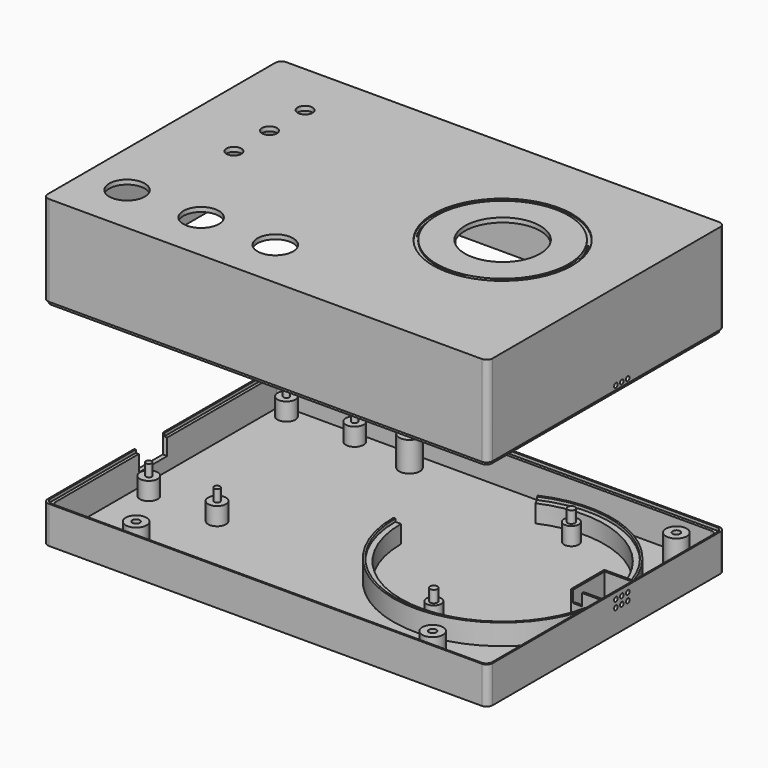
from build123d import *

# Parameters (mm, degrees)
F1_DEPTH  = 6
F0_R      = 2.5
F0_R_2    = 1.25
F0_R_3    = 3
F0_R_4    = 1
F0_W      = 3
F0_H      = 0.7
F2_DEPTH  = 10
F3_DEPTH  = 10
F0_R_5    = 3.5
F4_DEPTH  = 10
F5_DEPTH  = 4.5
F6_DEPTH  = 11
F7_DEPTH  = 7
F8_START  = 7.5
F8_DEPTH  = 2.5
F9_DEPTH  = 1.5
F10_R     = 2
F14_DEPTH = 30
F13_R     = 3.5
F15_DEPTH = 29
F13_R_2   = 2
F16_DEPTH = 7
F13_R_3   = 6
F13_R_4   = 2.5
F13_R_5   = 23.495
F17_DEPTH = 1.5
F13_R_6   = 12.7
F18_DEPTH = 1
F19_D     = 1.6
F19_DEPTH = 30.001
F20_D     = 1.6
F20_DEPTH = 30.001
F22_R     = 2
F23_DEPTH = 28
F24_DEPTH = 27
F26_R     = 0.75
F27_DEPTH = 1.5


# Not quite as in the source:
# - a feature of the source that left no trace in its solid (it failed there, or was rolled back) is left out
# - a feature names something its author has since deleted; it is built from what else it names


with BuildPart() as f1:
    # F0 (on Top) → F1 (new body)
    with BuildSketch(Plane.XY):
        with BuildLine():
            ThreePointArc((-14.0198845395, 31.2929215239), (15.59063064, 30.5407324118), (33.567902824, 7))
            Line((33.567902824, 7), (35.5116604089, 7))
            ThreePointArc((35.5116604089, 7), (16.6332395549, 32.1467473768), (-14.798767014, 33.0314171641))
            Line((-14.798767014, 33.0314171641), (-14.0198845395, 31.2929215239))
        make_face()
    extrude(amount=F1_DEPTH)



with BuildPart() as f1b:
    # F0 (on Top) → F1, piece 2 (new body)
    with BuildSketch(Plane.XY):
        with BuildLine():
            Line((-34.29, 0), (-36.195, 0))
            ThreePointArc((-36.195, 0), (-3.5166373497, -36.0237600307), (35.5116604089, -7))
            Line((35.5116604089, -7), (33.567902824, -7))
            ThreePointArc((33.567902824, -7), (-3.518573018, -34.1089979905), (-34.29, 0))
        make_face()
    extrude(amount=F1_DEPTH)


with BuildPart() as f1c:
    # F0 (on Top) → F1, piece 3 (new body)
    with BuildSketch(Plane.XY):
        with Locations((0, -29)):
            Circle(F0_R)
        with Locations((0, -29)):
            Circle(F0_R_2, mode=Mode.SUBTRACT)
    extrude(amount=F1_DEPTH)

    # F0 (on Top) → F2, piece 2 (join)
    with BuildSketch(Plane.XY):
        with Locations((0, -29)):
            Circle(F0_R_2)
    extrude(amount=F2_DEPTH)


with BuildPart() as f1d:
    # F0 (on Top) → F1, piece 4 (new body)
    with BuildSketch(Plane.XY):
        with Locations((0, 29)):
            Circle(F0_R)
        with Locations((0, 29)):
            Circle(F0_R_2, mode=Mode.SUBTRACT)
    extrude(amount=F1_DEPTH)

    # F0 (on Top) → F2 (join)
    with BuildSketch(Plane.XY):
        with Locations((0, 29)):
            Circle(F0_R_2)
    extrude(amount=F2_DEPTH)


with BuildPart() as f1e:
    # F0 (on Top) → F1, piece 5 (new body)
    with BuildSketch(Plane.XY):
        with Locations((-80.305, 38.0003526509)):
            Circle(F0_R_3)
        with Locations((-80.305, 38.0003526509)):
            Circle(F0_R_4, mode=Mode.SUBTRACT)
    extrude(amount=F1_DEPTH)

    # F0 (on Top) → F2, piece 4 (join)
    with BuildSketch(Plane.XY):
        with Locations((-80.305, 38.0003526509)):
            Circle(F0_R_4)
    extrude(amount=F2_DEPTH)


with BuildPart() as f1f:
    # F0 (on Top) → F1, piece 6 (new body)
    with BuildSketch(Plane.XY):
        with Locations((-103.305, 38.0003526509)):
            Circle(F0_R_3)
        with Locations((-103.305, 38.0003526509)):
            Circle(F0_R_4, mode=Mode.SUBTRACT)
    extrude(amount=F1_DEPTH)

    # F0 (on Top) → F2, piece 3 (join)
    with BuildSketch(Plane.XY):
        with Locations((-103.305, 38.0003526509)):
            Circle(F0_R_4)
    extrude(amount=F2_DEPTH)


with BuildPart() as f1g:
    # F0 (on Top) → F1, piece 7 (new body)
    with BuildSketch(Plane.XY):
        with Locations((-80.305, -19.9996473491)):
            Circle(F0_R_3)
        with Locations((-80.305, -19.9996473491)):
            Circle(F0_R_4, mode=Mode.SUBTRACT)
    extrude(amount=F1_DEPTH)

    # F0 (on Top) → F2, piece 5 (join)
    with BuildSketch(Plane.XY):
        with Locations((-80.305, -19.9996473491)):
            Circle(F0_R_4)
    extrude(amount=F2_DEPTH)


with BuildPart() as f1h:
    # F0 (on Top) → F1, piece 8 (new body)
    with BuildSketch(Plane.XY):
        with Locations((-103.305, -19.9996473491)):
            Circle(F0_R_3)
        with Locations((-103.305, -19.9996473491)):
            Circle(F0_R_4, mode=Mode.SUBTRACT)
    extrude(amount=F1_DEPTH)

    # F0 (on Top) → F2, piece 6 (join)
    with BuildSketch(Plane.XY):
        with Locations((-103.305, -19.9996473491)):
            Circle(F0_R_4)
    extrude(amount=F2_DEPTH)


with BuildPart() as f1i:
    # F0 (on Top) → F1, piece 9 (new body)
    with BuildSketch(Plane.XY):
        with Locations((30.895, -6.65)):
            Rectangle(F0_W, F0_H)
    extrude(amount=F1_DEPTH)


with BuildPart() as f1j:
    # F0 (on Top) → F1, piece 10 (new body)
    with BuildSketch(Plane.XY):
        Polygon((-96.805, 42.0003526509), (-82.805, 42.0003526509), (-82.805, 43.0003526509), (-82.805, 43.5003526509), (-96.805, 43.5003526509), (-96.805, 43.0003526509), align=None)
    extrude(amount=F1_DEPTH)


with BuildPart() as f1_1:
    add(f1.part)

    add(f1b.part)  # F3 merges F1b

    add(f1i.part)  # F3 merges F1i
    # F0 (on Top) → F3 (join)
    with BuildSketch(Plane.XY):
        Polygon((28.695, -7), (29.395, -7), (29.395, -6.3), (29.395, 6.3), (38.695, 6.3), (38.695, 7), (36.1586628624, 7), (35.5116604089, 7), (33.567902824, 7), (28.695, 7), align=None)
        Polygon((33.567902824, -7), (35.5116604089, -7), (36.1586628624, -7), (38.695, -7), (38.695, -6.3), (32.395, -6.3), (32.395, -7), align=None)
    extrude(amount=F3_DEPTH)


    add(f1j.part)  # F4 merges F1j
    # F0 (on Top) → F4 (join)
    with BuildSketch(Plane.XY):
        Polygon((38.695, -6.3), (38.695, -7), (38.695, -54.9996473491), (-108.305, -54.9996473491), (-108.305, -17.9996473491), (-109.305, -17.9996473491), (-109.305, -55.9996473491), (39.695, -55.9996473491), (39.695, 43.0003526509), (-82.805, 43.0003526509), (-82.805, 42.0003526509), (38.695, 42.0003526509), (38.695, 7), (38.695, 6.3), align=None)
        Polygon((-109.305, -5.9996473491), (-108.305, -5.9996473491), (-108.305, 42.0003526509), (-96.805, 42.0003526509), (-96.805, 43.0003526509), (-109.305, 43.0003526509), align=None)
    extrude(amount=F4_DEPTH)

    # F0 (on Top) → F5 (join)
    with BuildSketch(Plane.XY):
        Polygon((-109.305, -17.9996473491), (-108.305, -17.9996473491), (-108.305, -5.9996473491), (-109.305, -5.9996473491), (-109.805, -5.9996473491), (-109.805, -17.9996473491), align=None)
    extrude(amount=F5_DEPTH)

    # F0 (on Top) → F6 (join)
    with BuildSketch(Plane.XY):
        Polygon((-109.305, -55.9996473491), (-109.305, -17.9996473491), (-109.805, -17.9996473491), (-109.805, -56.4996473491), (40.195, -56.4996473491), (40.195, 43.5003526509), (-82.805, 43.5003526509), (-82.805, 43.0003526509), (39.695, 43.0003526509), (39.695, -55.9996473491), align=None)
        Polygon((-109.805, -5.9996473491), (-109.305, -5.9996473491), (-109.305, 43.0003526509), (-96.805, 43.0003526509), (-96.805, 43.5003526509), (-109.805, 43.5003526509), align=None)
    extrude(amount=F6_DEPTH)

    # F0 (on Top) → F7 (join)
    with BuildSketch(Plane.XY):
        with BuildLine():
            Line((35.5116604089, 7), (36.1586628624, 7))
            ThreePointArc((36.1586628624, 7), (16.9805930381, 32.6819271169), (-15.0583945054, 33.6109157108))
            Line((-15.0583945054, 33.6109157108), (-14.798767014, 33.0314171641))
            ThreePointArc((-14.798767014, 33.0314171641), (16.6332395549, 32.1467473768), (35.5116604089, 7))
        make_face()
        with BuildLine():
            ThreePointArc((35.5116604089, -7), (-3.5166373497, -36.0237600307), (-36.195, 0))
            Line((-36.195, 0), (-36.83, 0))
            ThreePointArc((-36.83, 0), (-3.516059355, -36.6617815526), (36.1586628624, -7))
            Line((36.1586628624, -7), (35.5116604089, -7))
        make_face()
    extrude(amount=F7_DEPTH)


    add(f1c.part)  # F9 merges F1c

    add(f1d.part)  # F9 merges F1d

    add(f1e.part)  # F9 merges F1e

    add(f1f.part)  # F9 merges F1f

    add(f1g.part)  # F9 merges F1g

    add(f1h.part)  # F9 merges F1h


with BuildPart() as f3:
    # F0 (on Top) → F3, piece 2 (new body)
    with BuildSketch(Plane.XY):
        with Locations((15.195, -48.4996473491)):
            Circle(F0_R_5)
        with Locations((15.195, -48.4996473491)):
            Circle(F0_R, mode=Mode.SUBTRACT)
    extrude(amount=F3_DEPTH)

    # F0 (on Top) → F8, piece 3 (join)
    with BuildSketch(Plane.XY.offset(F8_START)):
        with Locations((15.195, -48.4996473491)):
            Circle(F0_R)
        with Locations((15.195, -48.4996473491)):
            Circle(F0_R_2, mode=Mode.SUBTRACT)
    extrude(amount=F8_DEPTH)


with BuildPart() as f3b:
    # F0 (on Top) → F3, piece 3 (new body)
    with BuildSketch(Plane.XY):
        with Locations((30.195, 35.5003526509)):
            Circle(F0_R_5)
        with Locations((30.195, 35.5003526509)):
            Circle(F0_R, mode=Mode.SUBTRACT)
    extrude(amount=F3_DEPTH)

    # F0 (on Top) → F8, piece 4 (join)
    with BuildSketch(Plane.XY.offset(F8_START)):
        with Locations((30.195, 35.5003526509)):
            Circle(F0_R)
        with Locations((30.195, 35.5003526509)):
            Circle(F0_R_2, mode=Mode.SUBTRACT)
    extrude(amount=F8_DEPTH)


with BuildPart() as f3c:
    # F0 (on Top) → F3, piece 4 (new body)
    with BuildSketch(Plane.XY):
        with Locations((-84.805, -48.4996473491)):
            Circle(F0_R_5)
        with Locations((-84.805, -48.4996473491)):
            Circle(F0_R, mode=Mode.SUBTRACT)
    extrude(amount=F3_DEPTH)

    # F0 (on Top) → F8 (join)
    with BuildSketch(Plane.XY.offset(F8_START)):
        with Locations((-84.805, -48.4996473491)):
            Circle(F0_R)
        with Locations((-84.805, -48.4996473491)):
            Circle(F0_R_2, mode=Mode.SUBTRACT)
    extrude(amount=F8_DEPTH)


with BuildPart() as f3d:
    # F0 (on Top) → F3, piece 5 (new body)
    with BuildSketch(Plane.XY):
        with Locations((-59.805, 35.5003526509)):
            Circle(F0_R_5)
        with Locations((-59.805, 35.5003526509)):
            Circle(F0_R, mode=Mode.SUBTRACT)
    extrude(amount=F3_DEPTH)

    # F0 (on Top) → F8, piece 2 (join)
    with BuildSketch(Plane.XY.offset(F8_START)):
        with Locations((-59.805, 35.5003526509)):
            Circle(F0_R)
        with Locations((-59.805, 35.5003526509)):
            Circle(F0_R_2, mode=Mode.SUBTRACT)
    extrude(amount=F8_DEPTH)


with BuildPart() as f1_2:
    add(f1_1.part)

    add(f3.part)  # F9 merges F3

    add(f3b.part)  # F9 merges F3b

    add(f3c.part)  # F9 merges F3c

    add(f3d.part)  # F9 merges F3d
    # F0 (on Top) → F9 (join)
    with BuildSketch(Plane.XY):
        Polygon((-109.305, -55.9996473491), (-109.305, -17.9996473491), (-109.805, -17.9996473491), (-109.805, -56.4996473491), (40.195, -56.4996473491), (40.195, 43.5003526509), (-82.805, 43.5003526509), (-82.805, 43.0003526509), (39.695, 43.0003526509), (39.695, -55.9996473491), align=None)
        Polygon((38.695, -6.3), (38.695, -7), (38.695, -54.9996473491), (-108.305, -54.9996473491), (-108.305, -17.9996473491), (-109.305, -17.9996473491), (-109.305, -55.9996473491), (39.695, -55.9996473491), (39.695, 43.0003526509), (-82.805, 43.0003526509), (-82.805, 42.0003526509), (38.695, 42.0003526509), (38.695, 7), (38.695, 6.3), align=None)
        Polygon((-109.305, -17.9996473491), (-108.305, -17.9996473491), (-108.305, -5.9996473491), (-109.305, -5.9996473491), (-109.805, -5.9996473491), (-109.805, -17.9996473491), align=None)
        Polygon((-109.805, -5.9996473491), (-109.305, -5.9996473491), (-109.305, 43.0003526509), (-96.805, 43.0003526509), (-96.805, 43.5003526509), (-109.805, 43.5003526509), align=None)
        Polygon((-109.305, -5.9996473491), (-108.305, -5.9996473491), (-108.305, 42.0003526509), (-96.805, 42.0003526509), (-96.805, 43.0003526509), (-109.305, 43.0003526509), align=None)
        Polygon((-96.805, 42.0003526509), (-82.805, 42.0003526509), (-82.805, 43.0003526509), (-82.805, 43.5003526509), (-96.805, 43.5003526509), (-96.805, 43.0003526509), align=None)
        with BuildLine():
            Line((-36.83, 0), (-36.195, 0))
            Line((-36.195, 0), (-34.29, 0))
            ThreePointArc((-34.29, 0), (-3.518573018, -34.1089979905), (33.567902824, -7))
            Line((33.567902824, -7), (32.395, -7))
            Line((32.395, -7), (29.395, -7))
            Line((29.395, -7), (28.695, -7))
            Line((28.695, -7), (28.695, 7))
            Line((28.695, 7), (33.567902824, 7))
            ThreePointArc((33.567902824, 7), (15.59063064, 30.5407324118), (-14.0198845395, 31.2929215239))
            Line((-14.0198845395, 31.2929215239), (-14.798767014, 33.0314171641))
            Line((-14.798767014, 33.0314171641), (-15.0583945054, 33.6109157108))
            ThreePointArc((-15.0583945054, 33.6109157108), (16.9805930381, 32.6819271169), (36.1586628624, 7))
            Line((36.1586628624, 7), (38.695, 7))
            Line((38.695, 7), (38.695, 42.0003526509))
            Line((38.695, 42.0003526509), (-82.805, 42.0003526509))
            Line((-82.805, 42.0003526509), (-96.805, 42.0003526509))
            Line((-96.805, 42.0003526509), (-108.305, 42.0003526509))
            Line((-108.305, 42.0003526509), (-108.305, -5.9996473491))
            Line((-108.305, -5.9996473491), (-108.305, -17.9996473491))
            Line((-108.305, -17.9996473491), (-108.305, -54.9996473491))
            Line((-108.305, -54.9996473491), (38.695, -54.9996473491))
            Line((38.695, -54.9996473491), (38.695, -7))
            Line((38.695, -7), (36.1586628624, -7))
            ThreePointArc((36.1586628624, -7), (-3.516059355, -36.6617815526), (-36.83, 0))
        make_face()
        with Locations((-84.805, -48.4996473491)):
            Circle(F0_R_5, mode=Mode.SUBTRACT)
        with Locations((-103.305, -19.9996473491)):
            Circle(F0_R_3, mode=Mode.SUBTRACT)
        with Locations((-80.305, -19.9996473491)):
            Circle(F0_R_3, mode=Mode.SUBTRACT)
        with Locations((15.195, -48.4996473491)):
            Circle(F0_R_5, mode=Mode.SUBTRACT)
        with Locations((0, -29)):
            Circle(F0_R, mode=Mode.SUBTRACT)
        with Locations((-103.305, 38.0003526509)):
            Circle(F0_R_3, mode=Mode.SUBTRACT)
        with Locations((-80.305, 38.0003526509)):
            Circle(F0_R_3, mode=Mode.SUBTRACT)
        with Locations((-59.805, 35.5003526509)):
            Circle(F0_R_5, mode=Mode.SUBTRACT)
        with Locations((0, 29)):
            Circle(F0_R, mode=Mode.SUBTRACT)
        with Locations((30.195, 35.5003526509)):
            Circle(F0_R_5, mode=Mode.SUBTRACT)
        with Locations((-103.305, 38.0003526509)):
            Circle(F0_R_3)
        with Locations((-103.305, 38.0003526509)):
            Circle(F0_R_4, mode=Mode.SUBTRACT)
        with Locations((-103.305, 38.0003526509)):
            Circle(F0_R_4)
        with Locations((-80.305, 38.0003526509)):
            Circle(F0_R_3)
        with Locations((-80.305, 38.0003526509)):
            Circle(F0_R_4, mode=Mode.SUBTRACT)
        with Locations((-80.305, 38.0003526509)):
            Circle(F0_R_4)
        with Locations((-59.805, 35.5003526509)):
            Circle(F0_R_5)
        with Locations((-59.805, 35.5003526509)):
            Circle(F0_R, mode=Mode.SUBTRACT)
        with Locations((-84.805, -48.4996473491)):
            Circle(F0_R_5)
        with Locations((-84.805, -48.4996473491)):
            Circle(F0_R, mode=Mode.SUBTRACT)
        with Locations((-103.305, -19.9996473491)):
            Circle(F0_R_3)
        with Locations((-103.305, -19.9996473491)):
            Circle(F0_R_4, mode=Mode.SUBTRACT)
        with Locations((-103.305, -19.9996473491)):
            Circle(F0_R_4)
        with Locations((-80.305, -19.9996473491)):
            Circle(F0_R_3)
        with Locations((-80.305, -19.9996473491)):
            Circle(F0_R_4, mode=Mode.SUBTRACT)
        with Locations((-80.305, -19.9996473491)):
            Circle(F0_R_4)
        with Locations((0, 29)):
            Circle(F0_R)
        with Locations((0, 29)):
            Circle(F0_R_2, mode=Mode.SUBTRACT)
        with Locations((0, 29)):
            Circle(F0_R_2)
        with BuildLine():
            ThreePointArc((-14.0198845395, 31.2929215239), (15.59063064, 30.5407324118), (33.567902824, 7))
            Line((33.567902824, 7), (35.5116604089, 7))
            ThreePointArc((35.5116604089, 7), (16.6332395549, 32.1467473768), (-14.798767014, 33.0314171641))
            Line((-14.798767014, 33.0314171641), (-14.0198845395, 31.2929215239))
        make_face()
        with BuildLine():
            Line((35.5116604089, 7), (36.1586628624, 7))
            ThreePointArc((36.1586628624, 7), (16.9805930381, 32.6819271169), (-15.0583945054, 33.6109157108))
            Line((-15.0583945054, 33.6109157108), (-14.798767014, 33.0314171641))
            ThreePointArc((-14.798767014, 33.0314171641), (16.6332395549, 32.1467473768), (35.5116604089, 7))
        make_face()
        with BuildLine():
            Line((-34.29, 0), (-36.195, 0))
            ThreePointArc((-36.195, 0), (-3.5166373497, -36.0237600307), (35.5116604089, -7))
            Line((35.5116604089, -7), (33.567902824, -7))
            ThreePointArc((33.567902824, -7), (-3.518573018, -34.1089979905), (-34.29, 0))
        make_face()
        with BuildLine():
            ThreePointArc((35.5116604089, -7), (-3.5166373497, -36.0237600307), (-36.195, 0))
            Line((-36.195, 0), (-36.83, 0))
            ThreePointArc((-36.83, 0), (-3.516059355, -36.6617815526), (36.1586628624, -7))
            Line((36.1586628624, -7), (35.5116604089, -7))
        make_face()
        with Locations((30.195, 35.5003526509)):
            Circle(F0_R_5)
        with Locations((30.195, 35.5003526509)):
            Circle(F0_R, mode=Mode.SUBTRACT)
        Polygon((28.695, -7), (29.395, -7), (29.395, -6.3), (29.395, 6.3), (38.695, 6.3), (38.695, 7), (36.1586628624, 7), (35.5116604089, 7), (33.567902824, 7), (28.695, 7), align=None)
        Polygon((32.395, -6.3), (38.695, -6.3), (38.695, 6.3), (29.395, 6.3), (29.395, -6.3), align=None)
        Polygon((33.567902824, -7), (35.5116604089, -7), (36.1586628624, -7), (38.695, -7), (38.695, -6.3), (32.395, -6.3), (32.395, -7), align=None)
        with Locations((30.895, -6.65)):
            Rectangle(F0_W, F0_H)
        with Locations((0, -29)):
            Circle(F0_R)
        with Locations((0, -29)):
            Circle(F0_R_2, mode=Mode.SUBTRACT)
        with Locations((0, -29)):
            Circle(F0_R_2)
        with Locations((15.195, -48.4996473491)):
            Circle(F0_R_5)
        with Locations((15.195, -48.4996473491)):
            Circle(F0_R, mode=Mode.SUBTRACT)
    extrude(amount=-F9_DEPTH)

    # F10
    f10_edges = [f1_2.edges().sort_by_distance(p)[0] for p in [
        (38.695, 42.000353, 5),
        (39.695, 43.000353, 10.5),
        (40.195, 43.500353, 4.75),
        (40.195, -56.499647, 4.75),
        (38.695, -54.999647, 5),
        (39.695, -55.999647, 10.5),
        (-108.305, 42.000353, 5),
        (-109.305, 43.000353, 10.5),
        (-108.305, -54.999647, 5),
        (-109.305, -55.999647, 10.5),
        (-109.805, 43.500353, 4.75),
        (-109.805, -56.499647, 4.75),
    ]]
    fillet(f10_edges, radius=F10_R)


with BuildPart() as f14:
    # F13 (on offset) → F14 (new body)
    with BuildSketch(Plane.XY.offset(100)):
        Polygon((-109.305, 43.0003526509), (-109.305, -5.9996473491), (-108.305, -5.9996473491), (-108.305, 42.0003526509), (-96.805, 42.0003526509), (-96.805, 43.0003526509), align=None)
    extrude(amount=-F14_DEPTH)

    # F13 (on offset) → F15, piece 2 (join)
    with BuildSketch(Plane.XY.offset(100)):
        Polygon((-109.805, 43.5003526509), (-109.805, -5.9996473491), (-109.305, -5.9996473491), (-109.305, 43.0003526509), (-96.805, 43.0003526509), (-96.805, 43.5003526509), align=None)
    extrude(amount=-F15_DEPTH)



with BuildPart() as f14b:
    # F13 (on offset) → F14, piece 2 (new body)
    with BuildSketch(Plane.XY.offset(100)):
        with Locations((15.195, -48.4996473491)):
            Circle(F13_R)
    extrude(amount=-F14_DEPTH)


with BuildPart() as f14c:
    # F13 (on offset) → F14, piece 3 (new body)
    with BuildSketch(Plane.XY.offset(100)):
        with Locations((-84.805, -48.4996473491)):
            Circle(F13_R)
    extrude(amount=-F14_DEPTH)


with BuildPart() as f14d:
    # F13 (on offset) → F14, piece 4 (new body)
    with BuildSketch(Plane.XY.offset(100)):
        with Locations((-59.805, 35.5003526509)):
            Circle(F13_R)
    extrude(amount=-F14_DEPTH)


with BuildPart() as f14e:
    # F13 (on offset) → F14, piece 5 (new body)
    with BuildSketch(Plane.XY.offset(100)):
        with Locations((30.195, 35.5003526509)):
            Circle(F13_R)
    extrude(amount=-F14_DEPTH)


with BuildPart() as f14f:
    # F13 (on offset) → F14, piece 6 (new body)
    with BuildSketch(Plane.XY.offset(100)):
        Polygon((-108.305, -17.9996473491), (-109.305, -17.9996473491), (-109.305, -55.9996473491), (39.695, -55.9996473491), (39.695, 43.0003526509), (-82.805, 43.0003526509), (-82.805, 42.0003526509), (38.695, 42.0003526509), (38.695, -54.9996473491), (-108.305, -54.9996473491), align=None)
    extrude(amount=-F14_DEPTH)

    # F13 (on offset) → F15 (join)
    with BuildSketch(Plane.XY.offset(100)):
        Polygon((-109.805, -17.9996473491), (-109.805, -56.4996473491), (40.195, -56.4996473491), (40.195, 43.5003526509), (-82.805, 43.5003526509), (-82.805, 43.0003526509), (39.695, 43.0003526509), (39.695, -55.9996473491), (-109.305, -55.9996473491), (-109.305, -17.9996473491), align=None)
    extrude(amount=-F15_DEPTH)


with BuildPart() as f16:
    # F13 (on offset) → F16 (new body)
    with BuildSketch(Plane.XY.offset(100)):
        with Locations((18.415, 0)):
            Circle(F13_R_2)
    extrude(amount=-F16_DEPTH)



with BuildPart() as f16b:
    # F13 (on offset) → F16, piece 2 (new body)
    with BuildSketch(Plane.XY.offset(100)):
        with Locations((-18.415, 0)):
            Circle(F13_R_2)
    extrude(amount=-F16_DEPTH)


with BuildPart() as f14_1:
    add(f14.part)

    add(f14b.part)  # F17 merges F14b

    add(f14c.part)  # F17 merges F14c

    add(f14d.part)  # F17 merges F14d

    add(f14e.part)  # F17 merges F14e

    add(f14f.part)  # F17 merges F14f
    # F13 (on offset) → F17 (join)
    with BuildSketch(Plane.XY.offset(100)):
        Polygon((-109.805, -17.9996473491), (-109.805, -56.4996473491), (40.195, -56.4996473491), (40.195, 43.5003526509), (-82.805, 43.5003526509), (-82.805, 43.0003526509), (39.695, 43.0003526509), (39.695, -55.9996473491), (-109.305, -55.9996473491), (-109.305, -17.9996473491), align=None)
        Polygon((-109.305, 43.0003526509), (-109.305, -5.9996473491), (-108.305, -5.9996473491), (-108.305, 42.0003526509), (-96.805, 42.0003526509), (-96.805, 43.0003526509), align=None)
        Polygon((-108.305, -5.9996473491), (-108.305, -17.9996473491), (-108.305, -54.9996473491), (38.695, -54.9996473491), (38.695, 42.0003526509), (-82.805, 42.0003526509), (-96.805, 42.0003526509), (-108.305, 42.0003526509), align=None)
        with Locations((-84.805, -48.4996473491)):
            Circle(F13_R, mode=Mode.SUBTRACT)
        with Locations((-94.9426814914, -39.6566465497)):
            Circle(F13_R_3, mode=Mode.SUBTRACT)
        with Locations((-69.9426814914, -39.6566465497)):
            Circle(F13_R_3, mode=Mode.SUBTRACT)
        with Locations((-44.9426814914, -39.6566465497)):
            Circle(F13_R_3, mode=Mode.SUBTRACT)
        with Locations((15.195, -48.4996473491)):
            Circle(F13_R, mode=Mode.SUBTRACT)
        with Locations((-86.7926180363, -4.7786682844)):
            Circle(F13_R_4, mode=Mode.SUBTRACT)
        with Locations((-86.7926180363, 10.2213317156)):
            Circle(F13_R_4, mode=Mode.SUBTRACT)
        with Locations((-86.7926180363, 25.2213317156)):
            Circle(F13_R_4, mode=Mode.SUBTRACT)
        with Locations((-59.805, 35.5003526509)):
            Circle(F13_R, mode=Mode.SUBTRACT)
        Circle(F13_R_5, mode=Mode.SUBTRACT)
        with Locations((30.195, 35.5003526509)):
            Circle(F13_R, mode=Mode.SUBTRACT)
        with Locations((15.195, -48.4996473491)):
            Circle(F13_R)
        with Locations((-84.805, -48.4996473491)):
            Circle(F13_R)
        with Locations((30.195, 35.5003526509)):
            Circle(F13_R)
        with Locations((-59.805, 35.5003526509)):
            Circle(F13_R)
        Polygon((-82.805, 43.0003526509), (-82.805, 43.5003526509), (-96.805, 43.5003526509), (-96.805, 43.0003526509), (-96.805, 42.0003526509), (-82.805, 42.0003526509), align=None)
        Polygon((-109.805, -5.9996473491), (-109.805, -17.9996473491), (-109.305, -17.9996473491), (-108.305, -17.9996473491), (-108.305, -5.9996473491), (-109.305, -5.9996473491), align=None)
        Polygon((-108.305, -17.9996473491), (-109.305, -17.9996473491), (-109.305, -55.9996473491), (39.695, -55.9996473491), (39.695, 43.0003526509), (-82.805, 43.0003526509), (-82.805, 42.0003526509), (38.695, 42.0003526509), (38.695, -54.9996473491), (-108.305, -54.9996473491), align=None)
        Polygon((-109.805, 43.5003526509), (-109.805, -5.9996473491), (-109.305, -5.9996473491), (-109.305, 43.0003526509), (-96.805, 43.0003526509), (-96.805, 43.5003526509), align=None)
    extrude(amount=F17_DEPTH)



with BuildPart() as f16_1:
    add(f16.part)

    add(f16b.part)  # F17#2 merges F16b
    # F13 (on offset) → F17, piece 2 (join)
    with BuildSketch(Plane.XY.offset(100)):
        with BuildLine():
            ThreePointArc((11.7320383195, -18.8761728607), (19.4254366315, -10.7982885993), (22.225, 0))
            ThreePointArc((22.225, 0), (22.0928170025, 2.4203433421), (21.6978403245, 4.8118967415))
            ThreePointArc((21.6978403245, 4.8118967415), (20.579959338, 8.3914181546), (18.8761728607, 11.7320383195))
            ThreePointArc((18.8761728607, 11.7320383195), (8.6186001236, 20.4858574853), (-4.8118967415, 21.6978403245))
            ThreePointArc((-4.8118967415, 21.6978403245), (-8.3914181546, 20.579959338), (-11.7320383195, 18.8761728607))
            ThreePointArc((-11.7320383195, 18.8761728607), (-20.4858574853, 8.6186001236), (-21.6978403245, -4.8118967415))
            ThreePointArc((-21.6978403245, -4.8118967415), (-20.579959338, -8.3914181546), (-18.8761728607, -11.7320383195))
            ThreePointArc((-18.8761728607, -11.7320383195), (-8.6186001236, -20.4858574853), (4.8118967415, -21.6978403245))
            ThreePointArc((4.8118967415, -21.6978403245), (8.3914181546, -20.579959338), (11.7320383195, -18.8761728607))
        make_face()
        with Locations((-18.415, 0)):
            Circle(F13_R_2, mode=Mode.SUBTRACT)
        Circle(F13_R_6, mode=Mode.SUBTRACT)
        with Locations((18.415, 0)):
            Circle(F13_R_2, mode=Mode.SUBTRACT)
        with Locations((18.415, 0)):
            Circle(F13_R_2)
        with Locations((-18.415, 0)):
            Circle(F13_R_2)
    extrude(amount=F17_DEPTH)


with BuildPart() as f14_2:
    add(f14_1.part)

    add(f16_1.part)  # F18 merges F16
    # F13 (on offset) → F18 (join)
    with BuildSketch(Plane.XY.offset(100)):
        Circle(F13_R_5)
        with BuildLine():
            ThreePointArc((21.6978403245, 4.8118967415), (22.0928170025, 2.4203433421), (22.225, 0))
            ThreePointArc((22.225, 0), (19.4254366315, -10.7982885993), (11.7320383195, -18.8761728607))
            Line((11.7320383195, -18.8761728607), (12.0672394144, -19.4154920853))
            ThreePointArc((12.0672394144, -19.4154920853), (8.631172959, -21.1679581763), (4.9493795055, -22.3177786195))
            Line((4.9493795055, -22.3177786195), (4.8118967415, -21.6978403245))
            ThreePointArc((4.8118967415, -21.6978403245), (-8.6186001236, -20.4858574853), (-18.8761728607, -11.7320383195))
            Line((-18.8761728607, -11.7320383195), (-19.4154920853, -12.0672394144))
            ThreePointArc((-19.4154920853, -12.0672394144), (-21.1679581763, -8.631172959), (-22.3177786195, -4.9493795055))
            Line((-22.3177786195, -4.9493795055), (-21.6978403245, -4.8118967415))
            ThreePointArc((-21.6978403245, -4.8118967415), (-20.4858574853, 8.6186001236), (-11.7320383195, 18.8761728607))
            Line((-11.7320383195, 18.8761728607), (-12.0672394144, 19.4154920853))
            ThreePointArc((-12.0672394144, 19.4154920853), (-8.631172959, 21.1679581763), (-4.9493795055, 22.3177786195))
            Line((-4.9493795055, 22.3177786195), (-4.8118967415, 21.6978403245))
            ThreePointArc((-4.8118967415, 21.6978403245), (8.6186001236, 20.4858574853), (18.8761728607, 11.7320383195))
            Line((18.8761728607, 11.7320383195), (19.4154920853, 12.0672394144))
            ThreePointArc((19.4154920853, 12.0672394144), (21.1679581763, 8.631172959), (22.3177786195, 4.9493795055))
            Line((22.3177786195, 4.9493795055), (21.6978403245, 4.8118967415))
        make_face(mode=Mode.SUBTRACT)
    extrude(amount=F18_DEPTH)

    # F19 (through all, one way)
    with BuildSketch(Plane.XY.offset(100)):
        with Locations((-18.415, 0), (18.415, 0)):
            Circle(F19_D / 2)
    extrude(amount=-F19_DEPTH, mode=Mode.SUBTRACT)

    # F20 (through all, one way)
    with BuildSketch(Plane.XY.offset(100)):
        with Locations((-59.805, 35.5003526509), (30.195, 35.5003526509), (-84.805, -48.4996473491), (15.195, -48.4996473491)):
            Circle(F20_D / 2)
    extrude(amount=-F20_DEPTH, mode=Mode.SUBTRACT)

    # F21: union 

    # F22
    f22_edges = [f14_2.edges().sort_by_distance(p)[0] for p in [
        (-109.305, 43.000353, 70.5),
        (-109.305, -55.999647, 70.5),
        (39.695, -55.999647, 70.5),
        (39.695, 43.000353, 70.5),
        (38.695, -54.999647, 85),
        (38.695, 42.000353, 85),
        (-108.305, 42.000353, 85),
        (-108.305, -54.999647, 85),
        (-109.805, -56.499647, 86.25),
        (40.195, 43.500353, 86.25),
        (40.195, -56.499647, 86.25),
        (-109.805, 43.500353, 86.25),
    ]]
    fillet(f22_edges, radius=F22_R)

    # F13 (on offset) → F23 (join)
    with BuildSketch(Plane.XY.offset(100)):
        Polygon((-82.805, 43.0003526509), (-82.805, 43.5003526509), (-96.805, 43.5003526509), (-96.805, 43.0003526509), (-96.805, 42.0003526509), (-82.805, 42.0003526509), align=None)
    extrude(amount=-F23_DEPTH)

    # F13 (on offset) → F24 (join)
    with BuildSketch(Plane.XY.offset(100)):
        Polygon((-109.805, -5.9996473491), (-109.805, -17.9996473491), (-109.305, -17.9996473491), (-108.305, -17.9996473491), (-108.305, -5.9996473491), (-109.305, -5.9996473491), align=None)
    extrude(amount=-F24_DEPTH)


with BuildPart() as f27:
    # F26 (on offset) → F27 (new body)
    with BuildSketch(Plane.YZ.offset(40.195)):
        with Locations((-2.5, 8.8511314243)):
            Circle(F26_R)
    extrude(amount=-F27_DEPTH)


with BuildPart() as f27b:
    # F26 (on offset) → F27, piece 2 (new body)
    with BuildSketch(Plane.YZ.offset(40.195)):
        with Locations((0, 8.8511314243)):
            Circle(F26_R)
    extrude(amount=-F27_DEPTH)


with BuildPart() as f27c:
    # F26 (on offset) → F27, piece 3 (new body)
    with BuildSketch(Plane.YZ.offset(40.195)):
        with Locations((2.5, 8.8511314243)):
            Circle(F26_R)
    extrude(amount=-F27_DEPTH)


with BuildPart() as f27d:
    # F26 (on offset) → F27, piece 4 (new body)
    with BuildSketch(Plane.YZ.offset(40.195)):
        with Locations((-2.5, 6.3511314243)):
            Circle(F26_R)
    extrude(amount=-F27_DEPTH)


with BuildPart() as f27e:
    # F26 (on offset) → F27, piece 5 (new body)
    with BuildSketch(Plane.YZ.offset(40.195)):
        with Locations((0, 6.3511314243)):
            Circle(F26_R)
    extrude(amount=-F27_DEPTH)


with BuildPart() as f27f:
    # F26 (on offset) → F27, piece 6 (new body)
    with BuildSketch(Plane.YZ.offset(40.195)):
        with Locations((2.5, 6.3511314243)):
            Circle(F26_R)
    extrude(amount=-F27_DEPTH)


with BuildPart() as f27g:
    # F26 (on offset) → F27, piece 7 (new body)
    with BuildSketch(Plane.YZ.offset(40.195)):
        with Locations((-2.5, 72.3511314243)):
            Circle(F26_R)
    extrude(amount=-F27_DEPTH)


with BuildPart() as f27h:
    # F26 (on offset) → F27, piece 8 (new body)
    with BuildSketch(Plane.YZ.offset(40.195)):
        with Locations((0, 72.3511314243)):
            Circle(F26_R)
    extrude(amount=-F27_DEPTH)


with BuildPart() as f27i:
    # F26 (on offset) → F27, piece 9 (new body)
    with BuildSketch(Plane.YZ.offset(40.195)):
        with Locations((2.5, 72.3511314243)):
            Circle(F26_R)
    extrude(amount=-F27_DEPTH)


with BuildPart() as f1_3:
    add(f1_2.part)

    # F28: cut F27, F27d, F27e, F27f, F27b, F27c
    add(f27.part, mode=Mode.SUBTRACT)
    add(f27d.part, mode=Mode.SUBTRACT)
    add(f27e.part, mode=Mode.SUBTRACT)
    add(f27f.part, mode=Mode.SUBTRACT)
    add(f27b.part, mode=Mode.SUBTRACT)
    add(f27c.part, mode=Mode.SUBTRACT)


with BuildPart() as f14_3:
    add(f14_2.part)

    # F29: cut F27g, F27h, F27i
    add(f27g.part, mode=Mode.SUBTRACT)
    add(f27h.part, mode=Mode.SUBTRACT)
    add(f27i.part, mode=Mode.SUBTRACT)


solid = Compound([f1_3.part, f14_3.part])
